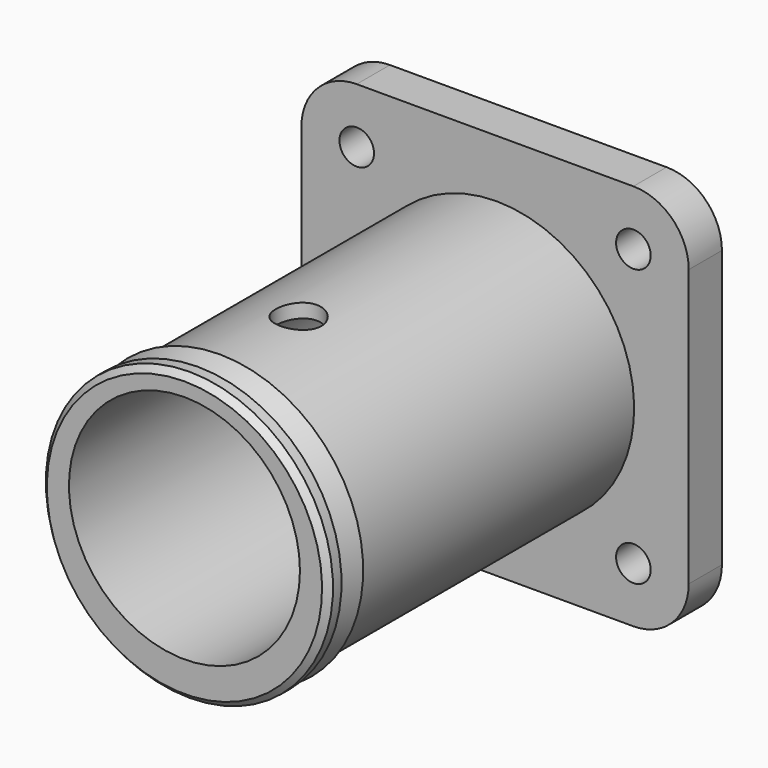
from build123d import *

# Parameters (mm, degrees)
F1_DEPTH  = 79.248
F3_DEPTH  = 11.2522
F6_R      = 3.175
F6_R_2    = 25.273
F6_R_3    = 21.209
F7_DEPTH  = 7.62
F9_R      = 4.191
F10_DEPTH = 7.874


# Not quite as in the source:
# - ends of sketch curves that miss each other by under 0.0002 mm in the source are joined
# - a feature names something its author has since deleted; it is built from what else it names


with BuildPart() as f1:
    # F0 (on Front) → F1 (new body)
    with BuildSketch(Plane.XZ):
        with BuildLine():
            ThreePointArc((25.2730608729, 1.6496396764), (17.870749032, 19.5203708791), (0, 26.9226396763))
            ThreePointArc((0, 26.9226396763), (-17.8706272863, -16.2210915263), (25.2730608729, 1.6496396764))
        make_face()
        with BuildLine():
            ThreePointArc((0, 24.3826396763), (14.9970630949, 18.1706867446), (21.2090547187, 3.1736396764))
            ThreePointArc((21.2090547187, 3.1736396764), (-14.9969536575, -11.8234073918), (0, 24.3826396763))
        make_face(mode=Mode.SUBTRACT)
    extrude(amount=-F1_DEPTH)

    # F2 (on face) → F3 (cut)
    with BuildSketch(Plane.XZ):
        with BuildLine():
            Line((24.13, 26.9226396763), (0, 26.9226396763))
            ThreePointArc((0, 26.9226396763), (8.7356829544, 25.3648971249), (16.3944827501, 20.8836579854))
            Line((16.3944827501, 20.8836579854), (24.13, 20.8835978808))
            Line((24.13, 20.8835978808), (24.13, 26.9226396763))
        make_face()
        with BuildLine():
            ThreePointArc((-16.3944315191, 20.8835978808), (-8.7356618013, 25.3648600709), (0, 26.9226396763))
            Line((0, 26.9226396763), (-24.13, 26.9226396763))
            Line((-24.13, 26.9226396763), (-24.13, 20.8835978808))
            Line((-24.13, 20.8835978808), (-16.3944315191, 20.8835978808))
        make_face()
    extrude(amount=-F3_DEPTH, mode=Mode.SUBTRACT)

    # F4 (on Right) → F5 (revolve)
    with BuildSketch(Plane.YZ):
        Polygon((1.143, 28.0148396764), (0, 26.9226396764), (3.0988, 26.9226396764), (3.0988, 28.0148396764), align=None)
        Polygon((8.0772, 28.0148396764), (3.0988, 26.9226396764), (8.0772, 26.9226396764), align=None)
    revolve(axis=Axis((6.08729e-05, 0, 1.6496396764), (0, 1, 0)))

    # F6 (on face) → F7 (join)
    with BuildSketch(Plane(origin=(0, 79.248, 0), x_dir=(-1, 0, 0), z_dir=(0, 1, 0))):
        with BuildLine():
            Line((-25.1332705243, -33.6252276427), (25.6667294757, -33.6252276427))
            ThreePointArc((25.6667294757, -33.6252276427), (32.8509343726, -30.6494325395), (35.8267294757, -23.4652276427))
            Line((35.8267294757, -23.4652276427), (35.8267294757, 27.3347723573))
            ThreePointArc((35.8267294757, 27.3347723573), (32.8509343726, 34.5189772542), (25.6667294757, 37.4947723573))
            Line((25.6667294757, 37.4947723573), (-25.1332705243, 37.4947723573))
            ThreePointArc((-25.1332705243, 37.4947723573), (-32.3174754212, 34.5189772542), (-35.2932705243, 27.3347723573))
            Line((-35.2932705243, 27.3347723573), (-35.2932705243, -23.4652276427))
            ThreePointArc((-35.2932705243, -23.4652276427), (-32.3174754212, -30.6494325395), (-25.1332705243, -33.6252276427))
        make_face()
        with Locations((-25.1332705243, -23.4652276427)):
            Circle(F6_R, mode=Mode.SUBTRACT)
        with Locations((-6.08729e-05, 1.6496396764)):
            Circle(F6_R_2, mode=Mode.SUBTRACT)
        with Locations((25.6667294757, -23.4652276427)):
            Circle(F6_R, mode=Mode.SUBTRACT)
        with Locations((-25.1332705243, 27.3347723573)):
            Circle(F6_R, mode=Mode.SUBTRACT)
        with Locations((25.6667294757, 27.3347723573)):
            Circle(F6_R, mode=Mode.SUBTRACT)
        with Locations((-6.08729e-05, 1.6496396764)):
            Circle(F6_R_2)
        with Locations((-5.47187e-05, 3.1736396764)):
            Circle(F6_R_3, mode=Mode.SUBTRACT)
    extrude(amount=-F7_DEPTH)

    # F9 (on offset) → F10 (cut)
    with BuildSketch(Plane.XY.offset(28.448)):
        with Locations((4.8756e-06, 26.1899903387)):
            Circle(F9_R)
    extrude(amount=-F10_DEPTH, mode=Mode.SUBTRACT)


solid = f1.part
